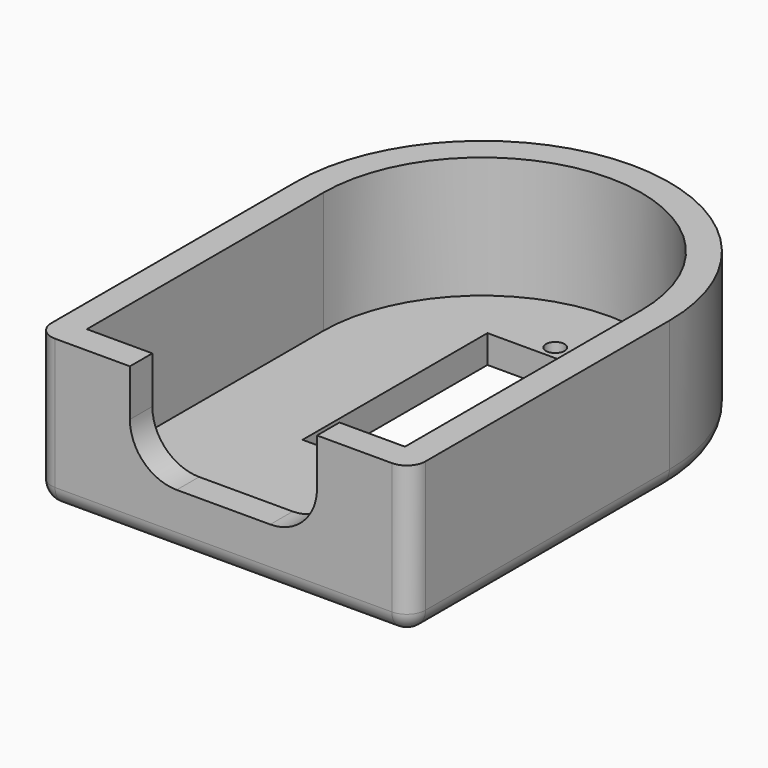
from build123d import *

# Parameters (mm, degrees)
F0_R     = 1
F1_DEPTH = 3
F2_DEPTH = 16
F3_R     = 2
F4_W     = 10
F4_H     = 10
F5_DEPTH = 3
F6_R     = 5


# Not quite as in the source:
# - a feature names something its author has since deleted; it is built from what else it names


with BuildPart() as f1:
    # F0 (on Top) → F1 (new body)
    with BuildSketch(Plane.XY):
        with BuildLine():
            Line((-10.95, 4.9143462471), (-10.95, 15.45))
            ThreePointArc((-10.95, 15.45), (6.05, 32.45), (23.05, 15.45))
            Line((23.05, 15.45), (23.05, 4.9143462471))
            ThreePointArc((23.05, 4.9143462471), (25.2853840617, 9.9727744249), (26.05, 15.45))
            ThreePointArc((26.05, 15.45), (6.05, 35.45), (-13.95, 15.45))
            ThreePointArc((-13.95, 15.45), (-13.1853840617, 9.9727744249), (-10.95, 4.9143462471))
        make_face()
        with BuildLine():
            Line((-10.95, -16.1332358822), (-10.95, 4.9143462471))
            ThreePointArc((-10.95, 4.9143462471), (-13.1853840617, 9.9727744249), (-13.95, 15.45))
            Line((-13.95, 15.45), (-13.95, -19.1332358822))
            Line((-13.95, -19.1332358822), (6.05, -19.1332358822))
            Line((6.05, -19.1332358822), (6.05, -16.1332358822))
            Line((6.05, -16.1332358822), (-10.95, -16.1332358822))
        make_face()
        with BuildLine():
            ThreePointArc((26.05, 15.45), (25.2853840617, 9.9727744249), (23.05, 4.9143462471))
            Line((23.05, 4.9143462471), (23.05, -16.1332358822))
            Line((23.05, -16.1332358822), (6.05, -16.1332358822))
            Line((6.05, -16.1332358822), (6.05, -19.1332358822))
            Line((6.05, -19.1332358822), (26.05, -19.1332358822))
            Line((26.05, -19.1332358822), (26.05, 15.45))
        make_face()
        with BuildLine():
            Line((0, 0), (0, 11.35))
            Line((0, 11.35), (-3, 11.35))
            Line((-3, 11.35), (-3, 1.0591174697))
            ThreePointArc((-3, 1.0591174697), (-1.5369696903, 0.2369171133), (0, -0.4370230062))
            Line((0, -0.4370230062), (0, 0))
        make_face()
        with BuildLine():
            Line((-3, -4.8), (-3, -2.3852880549))
            ThreePointArc((-3, -2.3852880549), (-7.4767065554, 0.7181226667), (-10.95, 4.9143462471))
            Line((-10.95, 4.9143462471), (-10.95, -16.1332358822))
            Line((-10.95, -16.1332358822), (6.05, -16.1332358822))
            Line((6.05, -16.1332358822), (6.05, -4.8))
            Line((6.05, -4.8), (-3, -4.8))
        make_face()
        with BuildLine():
            ThreePointArc((23.05, 4.9143462471), (19.5767065554, 0.7181226667), (15.1, -2.3852880549))
            Line((15.1, -2.3852880549), (15.1, -4.8))
            Line((15.1, -4.8), (6.05, -4.8))
            Line((6.05, -4.8), (6.05, -16.1332358822))
            Line((6.05, -16.1332358822), (23.05, -16.1332358822))
            Line((23.05, -16.1332358822), (23.05, 4.9143462471))
        make_face()
        with BuildLine():
            Line((-3, 1.0591174697), (-3, 11.35))
            Line((-3, 11.35), (-3, 27.5))
            Line((-3, 27.5), (15.1, 27.5))
            Line((15.1, 27.5), (15.1, 1.0591174697))
            ThreePointArc((15.1, 1.0591174697), (20.9303561785, 7.2295985499), (23.05, 15.45))
            ThreePointArc((23.05, 15.45), (6.05, 32.45), (-10.95, 15.45))
            ThreePointArc((-10.95, 15.45), (-8.8303561785, 7.2295985499), (-3, 1.0591174697))
        make_face()
        with BuildLine():
            ThreePointArc((23.05, 15.45), (20.9303561785, 7.2295985499), (15.1, 1.0591174697))
            Line((15.1, 1.0591174697), (15.1, -2.3852880549))
            ThreePointArc((15.1, -2.3852880549), (19.5767065554, 0.7181226667), (23.05, 4.9143462471))
            Line((23.05, 4.9143462471), (23.05, 15.45))
        make_face()
        with BuildLine():
            Line((-3, -2.3852880549), (-3, 1.0591174697))
            ThreePointArc((-3, 1.0591174697), (-8.8303561785, 7.2295985499), (-10.95, 15.45))
            Line((-10.95, 15.45), (-10.95, 4.9143462471))
            ThreePointArc((-10.95, 4.9143462471), (-7.4767065554, 0.7181226667), (-3, -2.3852880549))
        make_face()
        with BuildLine():
            Line((0, -1), (0, -0.4370230062))
            ThreePointArc((0, -0.4370230062), (-1.5369696903, 0.2369171133), (-3, 1.0591174697))
            Line((-3, 1.0591174697), (-3, -2.3852880549))
            ThreePointArc((-3, -2.3852880549), (1.3973535003, -4.0012950867), (6.05, -4.55))
            Line((6.05, -4.55), (6.05, -3.5))
            ThreePointArc((6.05, -3.5), (5.0618917373, -2.6537597518), (5.7461374375, -1.5472841226))
            ThreePointArc((5.7461374375, -1.5472841226), (3.7372080924, -1.3919415031), (1.7607692997, -1))
            Line((1.7607692997, -1), (0, -1))
        make_face()
        with BuildLine():
            ThreePointArc((6.05, -4.55), (1.3973535003, -4.0012950867), (-3, -2.3852880549))
            Line((-3, -2.3852880549), (-3, -4.8))
            Line((-3, -4.8), (6.05, -4.8))
            Line((6.05, -4.8), (6.05, -4.55))
        make_face()
        with BuildLine():
            Line((15.1, -4.8), (15.1, -2.3852880549))
            ThreePointArc((15.1, -2.3852880549), (10.7026464997, -4.0012950867), (6.05, -4.55))
            Line((6.05, -4.55), (6.05, -4.8))
            Line((6.05, -4.8), (15.1, -4.8))
        make_face()
        with BuildLine():
            ThreePointArc((15.1, 1.0591174697), (13.6369696903, 0.2369171133), (12.1, -0.4370230062))
            Line((12.1, -0.4370230062), (12.1, -1))
            Line((12.1, -1), (10.3392307003, -1))
            ThreePointArc((10.3392307003, -1), (8.3627919076, -1.3919415031), (6.3538625625, -1.5472841226))
            ThreePointArc((6.3538625625, -1.5472841226), (6.8574226163, -1.9100265101), (7.05, -2.5))
            ThreePointArc((7.05, -2.5), (6.7571067812, -3.2071067812), (6.05, -3.5))
            Line((6.05, -3.5), (6.05, -4.55))
            ThreePointArc((6.05, -4.55), (10.7026464997, -4.0012950867), (15.1, -2.3852880549))
            Line((15.1, -2.3852880549), (15.1, 1.0591174697))
        make_face()
        with BuildLine():
            Line((10.3392307003, -1), (6.05, -1))
            Line((6.05, -1), (6.05, -1.5))
            ThreePointArc((6.05, -1.5), (6.2037597518, -1.5118917373), (6.3538625625, -1.5472841226))
            ThreePointArc((6.3538625625, -1.5472841226), (8.3627919076, -1.3919415031), (10.3392307003, -1))
        make_face()
        with BuildLine():
            Line((6.05, -1.5), (6.05, -1))
            Line((6.05, -1), (1.7607692997, -1))
            ThreePointArc((1.7607692997, -1), (3.7372080924, -1.3919415031), (5.7461374375, -1.5472841226))
            ThreePointArc((5.7461374375, -1.5472841226), (5.8962402482, -1.5118917373), (6.05, -1.5))
        make_face()
        with BuildLine():
            Line((0, 11.35), (0, 22.7))
            Line((0, 22.7), (0, 23.7))
            Line((0, 23.7), (12.1, 23.7))
            Line((12.1, 23.7), (12.1, 22.7))
            Line((12.1, 22.7), (12.1, 0))
            Line((12.1, 0), (12.1, -0.4370230062))
            ThreePointArc((12.1, -0.4370230062), (13.6369696903, 0.2369171133), (15.1, 1.0591174697))
            Line((15.1, 1.0591174697), (15.1, 27.5))
            Line((15.1, 27.5), (-3, 27.5))
            Line((-3, 27.5), (-3, 11.35))
            Line((-3, 11.35), (0, 11.35))
        make_face()
        with Locations((6.05, 25.2)):
            Circle(F0_R, mode=Mode.SUBTRACT)
    extrude(amount=F1_DEPTH)

    # F0 (on Top) → F2 (join)
    with BuildSketch(Plane.XY):
        with BuildLine():
            Line((-10.95, -16.1332358822), (-10.95, 4.9143462471))
            ThreePointArc((-10.95, 4.9143462471), (-13.1853840617, 9.9727744249), (-13.95, 15.45))
            Line((-13.95, 15.45), (-13.95, -19.1332358822))
            Line((-13.95, -19.1332358822), (6.05, -19.1332358822))
            Line((6.05, -19.1332358822), (6.05, -16.1332358822))
            Line((6.05, -16.1332358822), (-10.95, -16.1332358822))
        make_face()
        with BuildLine():
            ThreePointArc((26.05, 15.45), (25.2853840617, 9.9727744249), (23.05, 4.9143462471))
            Line((23.05, 4.9143462471), (23.05, -16.1332358822))
            Line((23.05, -16.1332358822), (6.05, -16.1332358822))
            Line((6.05, -16.1332358822), (6.05, -19.1332358822))
            Line((6.05, -19.1332358822), (26.05, -19.1332358822))
            Line((26.05, -19.1332358822), (26.05, 15.45))
        make_face()
        with BuildLine():
            Line((-10.95, 4.9143462471), (-10.95, 15.45))
            ThreePointArc((-10.95, 15.45), (6.05, 32.45), (23.05, 15.45))
            Line((23.05, 15.45), (23.05, 4.9143462471))
            ThreePointArc((23.05, 4.9143462471), (25.2853840617, 9.9727744249), (26.05, 15.45))
            ThreePointArc((26.05, 15.45), (6.05, 35.45), (-13.95, 15.45))
            ThreePointArc((-13.95, 15.45), (-13.1853840617, 9.9727744249), (-10.95, 4.9143462471))
        make_face()
    extrude(amount=F2_DEPTH)

    # F3
    f3_edges = [f1.edges().sort_by_distance(p)[0] for p in [
        (26.05, -1.841618, 0),
        (-13.95, -1.841618, 0),
        (6.05, -19.133236, 0),
        (26.05, -19.133236, 8),
        (-13.95, -19.133236, 8),
    ]]
    fillet(f3_edges, radius=F3_R)

    # F4 (on face) → F5 (cut, through all)
    with BuildSketch(Plane.XZ.offset(19.1332358822)):
        with Locations((1.05, 11)):
            Rectangle(F4_W, F4_H)
        with Locations((11.05, 11)):
            Rectangle(F4_W, F4_H)
    extrude(amount=-F5_DEPTH, mode=Mode.SUBTRACT)

    # F6
    f6_edges = [f1.edges().sort_by_distance(p)[0] for p in [
        (-3.95, -17.633236, 6),
        (16.05, -17.633236, 6),
    ]]
    fillet(f6_edges, radius=F6_R)


solid = f1.part
